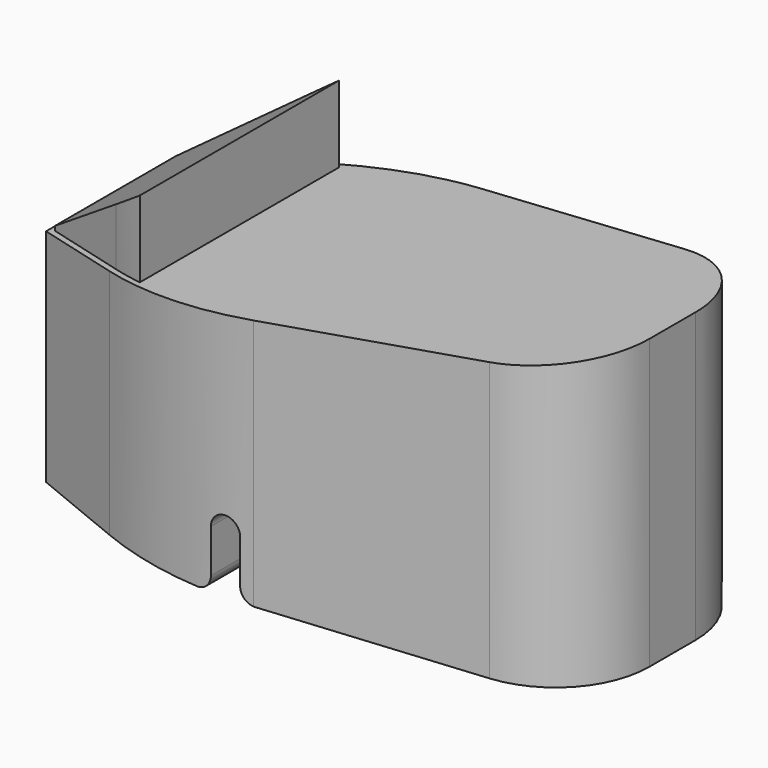
from build123d import *

# Parameters (mm, degrees)
F1_DEPTH  = 200
F4_DEPTH  = 110
F5_W      = 20
F5_H      = 50
F6_DEPTH  = 110
F7_R      = 10
F7_R_2    = 9.99999
F8_R      = 10
F12_DEPTH = 100


# Not quite as in the source:
# - a fillet or chamfer is up to 0.001 mm smaller than in the source, because OpenCascade refuses the exact size


with BuildPart() as f1:
    # F0 (on Top) → F1 (new body)
    with BuildSketch(Plane.XY):
        with BuildLine():
            Line((-129.7011448747, 82.0831308431), (-195, 55.2543373544))
            Line((-195, 55.2543373544), (-195, 0.2543373544))
            Line((-195, 0.2543373544), (195, 0.2543373544))
            Line((195, 0.2543373544), (195, 20.2543373544))
            ThreePointArc((195, 20.2543373544), (178.031605372, 64.0489133357), (135.9856958342, 84.9781463073))
            Line((135.9856958342, 84.9781463073), (-16.3916033039, 99.0700883522))
            ThreePointArc((-16.3916033039, 99.0700883522), (-74.0749348766, 97.4375057422), (-129.7011448747, 82.0831308431))
        make_face()
        with BuildLine():
            Line((195, 0.2543373544), (-195, 0.2543373544))
            Line((-195, 0.2543373544), (-195, -54.7456626456))
            Line((-195, -54.7456626456), (-129.7011448747, -81.5744561343))
            ThreePointArc((-129.7011448747, -81.5744561343), (-74.0749348766, -96.9288310334), (-16.3916033039, -98.5614136434))
            Line((-16.3916033039, -98.5614136434), (135.9856958342, -84.4694715986))
            ThreePointArc((135.9856958342, -84.4694715986), (178.031605372, -63.540238627), (195, -19.7456626456))
            Line((195, -19.7456626456), (195, 0.2543373544))
        make_face()
    extrude(amount=F1_DEPTH)

    # F3 (on Front) → F4 (cut, symmetric)
    with BuildSketch(Plane.XZ):
        Polygon((195, 200), (-195, 200), (-195, 153), align=None)
    extrude(amount=F4_DEPTH, both=True, mode=Mode.SUBTRACT)

    # F5 (on Front) → F6 (cut, symmetric)
    with BuildSketch(Plane.XZ):
        with Locations((-35, 25)):
            Rectangle(F5_W, F5_H)
    extrude(amount=F6_DEPTH, both=True, mode=Mode.SUBTRACT)

    # F7 (call 1 of 2: OpenCascade refuses the feature's edges together)
    f7_edges = [f1.edges().sort_by_distance(p)[0] for p in [
        (-25, 0.254337, 50),
    ]]
    fillet(f7_edges, radius=F7_R)

    # F7#2 (call 2 of 2) (radius 10 in the source; OpenCascade refuses exactly that, so slightly less here)
    f7_2_edges = [f1.edges().sort_by_distance(p)[0] for p in [
        (-45, 0.254337, 50),
    ]]
    fillet(f7_2_edges, radius=F7_R_2)

    # F8
    f8_edges = [f1.edges().sort_by_distance(p)[0] for p in [
        (-45, 0.254337, 0),
        (-25, 0.254337, 0),
    ]]
    fillet(f8_edges, radius=F8_R)

    # F9 (on offset) → F10 (join, up to the next surface of F1)
    with BuildSketch(Plane.XY.offset(220)):
        with BuildLine():
            Line((-105, -86.0161099703), (-105, 86.5247846791))
            ThreePointArc((-105, 86.5247846791), (-116.6965219134, 82.7558804952), (-128.181003028, 78.3832431737))
            Line((-128.181003028, 78.3832431737), (-191, 52.5733282266))
            Line((-191, 52.5733282266), (-191, -52.0646535178))
            Line((-191, -52.0646535178), (-128.181003028, -77.8745684649))
            ThreePointArc((-128.181003028, -77.8745684649), (-116.6965219134, -82.2472057865), (-105, -86.0161099703))
        make_face()
    extrude(until=Until.NEXT, dir=(0, 0, -1))

    # F11 (on Front) → F12 (cut, symmetric)
    with BuildSketch(Plane.XZ):
        Polygon((-191, 156.5037577633), (-105, 216.8246032937), (-105, 220), (-191, 220), align=None)
    extrude(amount=F12_DEPTH, both=True, mode=Mode.SUBTRACT)


solid = f1.part
